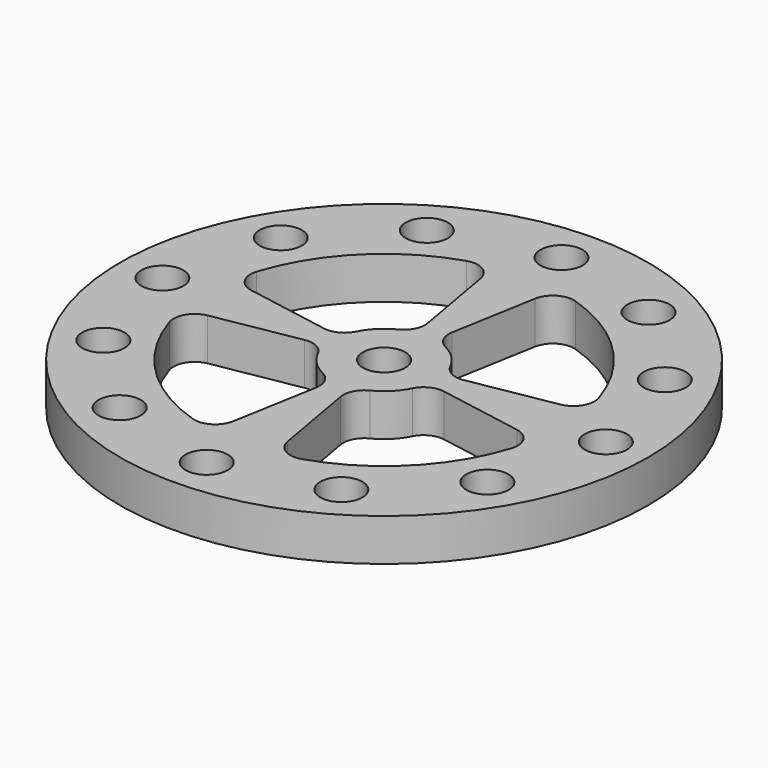
from build123d import *

# Parameters (mm, degrees)
F0_R     = 25
F0_R_2   = 2
F1_DEPTH = 4
F3_DEPTH = 25
F4_DEPTH = 25


# Not quite as in the source:
# - a feature names something its author has since deleted; it is built from what else it names


with BuildPart() as f1:
    # F0 (on Top) → F1 (new body)
    with BuildSketch(Plane.XY):
        Circle(F0_R)
        with Locations((-10.5, -18.1865334795)):
            Circle(F0_R_2, mode=Mode.SUBTRACT)
        with Locations((-18.1865334795, -10.5)):
            Circle(F0_R_2, mode=Mode.SUBTRACT)
        with Locations((0, -21)):
            Circle(F0_R_2, mode=Mode.SUBTRACT)
        with Locations((10.5, -18.1865334795)):
            Circle(F0_R_2, mode=Mode.SUBTRACT)
        with Locations((18.1865334795, -10.5)):
            Circle(F0_R_2, mode=Mode.SUBTRACT)
        with Locations((-21, 0)):
            Circle(F0_R_2, mode=Mode.SUBTRACT)
        with Locations((-18.1865334795, 10.5)):
            Circle(F0_R_2, mode=Mode.SUBTRACT)
        with Locations((-10.5, 18.1865334795)):
            Circle(F0_R_2, mode=Mode.SUBTRACT)
        Circle(F0_R_2, mode=Mode.SUBTRACT)
        with Locations((21, 0)):
            Circle(F0_R_2, mode=Mode.SUBTRACT)
        with Locations((18.1865334795, 10.5)):
            Circle(F0_R_2, mode=Mode.SUBTRACT)
        with Locations((10.5, 18.1865334795)):
            Circle(F0_R_2, mode=Mode.SUBTRACT)
        with Locations((0, 21)):
            Circle(F0_R_2, mode=Mode.SUBTRACT)
    extrude(amount=-F1_DEPTH)

    # F2 (on face) → F3 (cut)
    with BuildSketch(Plane.XY):
        with BuildLine():
            ThreePointArc((4.470710633, 2.2389163531), (5.3603810508, 1.3477279657), (6.6062912415, 1.1648673883))
            Line((6.6062912415, 1.1648673883), (14.6402197592, 2.581465747))
            ThreePointArc((14.6402197592, 2.581465747), (16.0042145423, 3.5159567971), (16.1986465243, 5.1578920868))
            ThreePointArc((16.1986465243, 5.1578920868), (12.0208152802, 12.0208152802), (5.1578920868, 16.1986465243))
            ThreePointArc((5.1578920868, 16.1986465243), (3.5159567971, 16.0042145423), (2.581465747, 14.6402197592))
            Line((2.581465747, 14.6402197592), (1.1648673883, 6.6062912415))
            ThreePointArc((1.1648673883, 6.6062912415), (1.3477279657, 5.3603810508), (2.2389163531, 4.470710633))
            ThreePointArc((2.2389163531, 4.470710633), (3.5355339059, 3.5355339059), (4.470710633, 2.2389163531))
        make_face()
        with BuildLine():
            ThreePointArc((-4.470710633, -2.2389163531), (-5.3603810508, -1.3477279657), (-6.6062912415, -1.1648673883))
            Line((-6.6062912415, -1.1648673883), (-14.6402197592, -2.581465747))
            ThreePointArc((-14.6402197592, -2.581465747), (-16.0042145423, -3.5159567971), (-16.1986465243, -5.1578920868))
            ThreePointArc((-16.1986465243, -5.1578920868), (-12.0208152802, -12.0208152802), (-5.1578920868, -16.1986465243))
            ThreePointArc((-5.1578920868, -16.1986465243), (-3.5159567971, -16.0042145423), (-2.581465747, -14.6402197592))
            Line((-2.581465747, -14.6402197592), (-1.1648673883, -6.6062912415))
            ThreePointArc((-1.1648673883, -6.6062912415), (-1.3477279657, -5.3603810508), (-2.2389163531, -4.470710633))
            ThreePointArc((-2.2389163531, -4.470710633), (-3.5355339059, -3.5355339059), (-4.470710633, -2.2389163531))
        make_face()
        with BuildLine():
            ThreePointArc((2.2389163531, -4.470710633), (1.3477279657, -5.3603810508), (1.1648673883, -6.6062912415))
            Line((1.1648673883, -6.6062912415), (2.581465747, -14.6402197592))
            ThreePointArc((2.581465747, -14.6402197592), (3.5159567971, -16.0042145423), (5.1578920868, -16.1986465243))
            ThreePointArc((5.1578920868, -16.1986465243), (12.0208152802, -12.0208152802), (16.1986465243, -5.1578920868))
            ThreePointArc((16.1986465243, -5.1578920868), (16.0042145423, -3.5159567971), (14.6402197592, -2.581465747))
            Line((14.6402197592, -2.581465747), (6.6062912415, -1.1648673883))
            ThreePointArc((6.6062912415, -1.1648673883), (5.3603810508, -1.3477279657), (4.470710633, -2.2389163531))
            ThreePointArc((4.470710633, -2.2389163531), (3.5355339059, -3.5355339059), (2.2389163531, -4.470710633))
        make_face()
    extrude(amount=-F3_DEPTH, mode=Mode.SUBTRACT)

    # F2 (on face) → F4 (cut)
    with BuildSketch(Plane.XY):
        with BuildLine():
            ThreePointArc((-2.581465747, 14.6402197592), (-3.5159567971, 16.0042145423), (-5.1578920868, 16.1986465243))
            ThreePointArc((-5.1578920868, 16.1986465243), (-12.0208152802, 12.0208152802), (-16.1986465243, 5.1578920868))
            ThreePointArc((-16.1986465243, 5.1578920868), (-16.0042145423, 3.5159567971), (-14.6402197592, 2.581465747))
            Line((-14.6402197592, 2.581465747), (-6.6062912415, 1.1648673883))
            ThreePointArc((-6.6062912415, 1.1648673883), (-5.3603810508, 1.3477279657), (-4.470710633, 2.2389163531))
            ThreePointArc((-4.470710633, 2.2389163531), (-3.5355339059, 3.5355339059), (-2.2389163531, 4.470710633))
            ThreePointArc((-2.2389163531, 4.470710633), (-1.3477279657, 5.3603810508), (-1.1648673883, 6.6062912415))
            Line((-1.1648673883, 6.6062912415), (-2.581465747, 14.6402197592))
        make_face()
    extrude(amount=-F4_DEPTH, mode=Mode.SUBTRACT)


solid = f1.part
